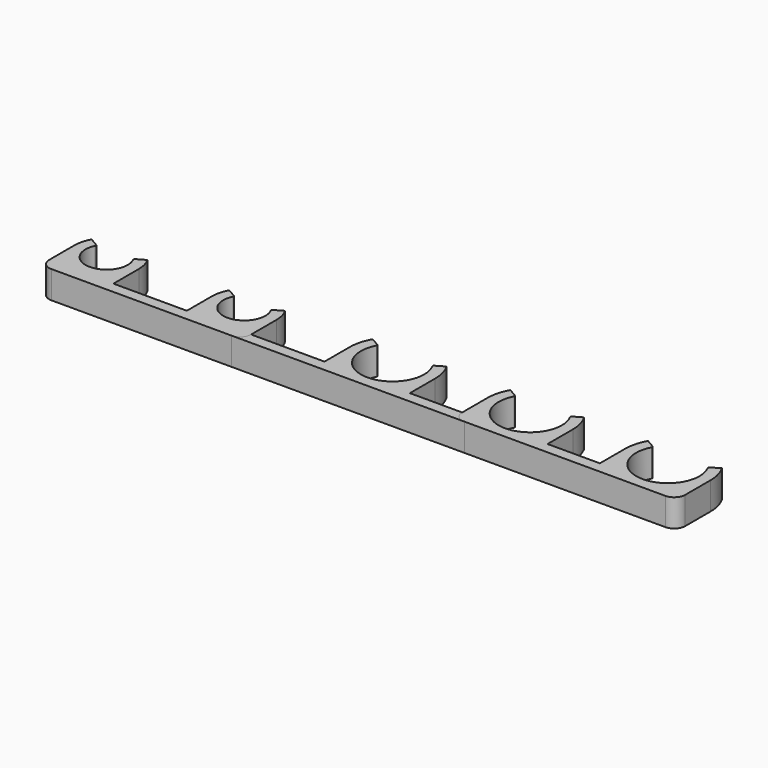
from build123d import *

# Parameters (mm, degrees)
F1_DEPTH = 5
F2_DEPTH = 5


# Not quite as in the source:
# - a feature names something its author has since deleted; it is built from what else it names


with BuildPart() as f1:
    # F0 (on Top) → F1 (new body)
    with BuildSketch(Plane.XY):
        with BuildLine():
            ThreePointArc((5.0906607601, 2.6735132364), (0, -5.75), (-5.0906607601, 2.6735132364))
            ThreePointArc((-5.0906607601, 2.6735132364), (-5.0718550548, 2.8592753519), (-5.1869938367, 3.0062592933))
            Line((-5.1869938367, 3.0062592933), (-6.7066912921, 3.8836570282))
            ThreePointArc((-6.7066912921, 3.8836570282), (-7.4846295003, 2.0106768122), (-7.75, 0))
            ThreePointArc((-7.75, 0), (-5.4800775542, -5.4800775542), (0, -7.75))
            ThreePointArc((0, -7.75), (5.4800775542, -5.4800775542), (7.75, 0))
            ThreePointArc((7.75, 0), (7.4846295003, 2.0106768122), (6.7066912921, 3.8836570282))
            Line((6.7066912921, 3.8836570282), (5.1869938367, 3.0062592933))
            ThreePointArc((5.1869938367, 3.0062592933), (5.0718550548, 2.8592753519), (5.0906607601, 2.6735132364))
        make_face()
        with BuildLine():
            ThreePointArc((0, -7.75), (-5.4800775542, -5.4800775542), (-7.75, 0))
            Line((-7.75, 0), (-7.75, -5.75))
            Line((-7.75, -5.75), (-21.075, -5.75))
            ThreePointArc((-21.075, -5.75), (-21.6607864376, -7.1642135624), (-23.075, -7.75))
            Line((-23.075, -7.75), (-7.75, -7.75))
            Line((-7.75, -7.75), (-5.75, -7.75))
            Line((-5.75, -7.75), (0, -7.75))
        make_face()
        with BuildLine():
            Line((7.75, -5.75), (7.75, 0))
            ThreePointArc((7.75, 0), (5.4800775542, -5.4800775542), (0, -7.75))
            Line((0, -7.75), (5.75, -7.75))
            Line((5.75, -7.75), (19.25, -7.75))
            ThreePointArc((19.25, -7.75), (17.8357864376, -7.1642135624), (17.25, -5.75))
            Line((17.25, -5.75), (7.75, -5.75))
        make_face()
    extrude(amount=F1_DEPTH)


with BuildPart() as f2:
    # F0 (on Top) → F2 (new body)
    with BuildSketch(Plane.XY):
        with BuildLine():
            ThreePointArc((-57.75, 0), (-51.9125, -5.8375), (-46.075, 0))
            ThreePointArc((-46.075, 0), (-46.2757134574, 1.5175782427), (-46.8640513825, 2.9307972987))
            Line((-46.8640513825, 2.9307972987), (-48.3854905692, 2.0523939747))
            ThreePointArc((-48.3854905692, 2.0523939747), (-48.5000018905, 1.9075418417), (-48.4838550604, 1.723600919))
            ThreePointArc((-48.4838550604, 1.723600919), (-51.9048651488, -3.8374924051), (-55.3479761214, 1.7099444637))
            ThreePointArc((-55.3479761214, 1.7099444637), (-55.3324173522, 1.8934720901), (-55.4467856407, 2.0378478482))
            Line((-55.4467856407, 2.0378478482), (-56.9690803045, 2.9167450821))
            ThreePointArc((-56.9690803045, 2.9167450821), (-57.5513914592, 1.5097381764), (-57.75, 0))
        make_face()
        with BuildLine():
            Line((-55.75, -7.75), (-48.075, -7.75))
            ThreePointArc((-48.075, -7.75), (-46.6607864376, -7.1642135624), (-46.075, -5.75))
            Line((-46.075, -5.75), (-46.075, 0))
            ThreePointArc((-46.075, 0), (-51.9125, -5.8375), (-57.75, 0))
            Line((-57.75, 0), (-57.75, -5.75))
            ThreePointArc((-57.75, -5.75), (-57.1642135624, -7.1642135624), (-55.75, -7.75))
        make_face()
        with BuildLine():
            ThreePointArc((-32.75, 0), (-26.9125, -5.8375), (-21.075, 0))
            ThreePointArc((-21.075, 0), (-21.2757134574, 1.5175782427), (-21.8640513825, 2.9307972987))
            Line((-21.8640513825, 2.9307972987), (-23.3854905692, 2.0523939747))
            ThreePointArc((-23.3854905692, 2.0523939747), (-23.5000018905, 1.9075418417), (-23.4838550604, 1.723600919))
            ThreePointArc((-23.4838550604, 1.723600919), (-26.9048651488, -3.8374924051), (-30.3479761214, 1.7099444637))
            ThreePointArc((-30.3479761214, 1.7099444637), (-30.3324173522, 1.8934720901), (-30.4467856407, 2.0378478482))
            Line((-30.4467856407, 2.0378478482), (-31.9690803045, 2.9167450821))
            ThreePointArc((-31.9690803045, 2.9167450821), (-32.5513914592, 1.5097381764), (-32.75, 0))
        make_face()
        with BuildLine():
            ThreePointArc((-23.075, -7.75), (-21.6607864376, -7.1642135624), (-21.075, -5.75))
            Line((-21.075, -5.75), (-21.075, 0))
            ThreePointArc((-21.075, 0), (-26.9125, -5.8375), (-32.75, 0))
            Line((-32.75, 0), (-32.75, -5.75))
            ThreePointArc((-32.75, -5.75), (-32.1642135624, -7.1642135624), (-30.75, -7.75))
            Line((-30.75, -7.75), (-23.075, -7.75))
        make_face()
        with BuildLine():
            Line((-48.075, -7.75), (-30.75, -7.75))
            ThreePointArc((-30.75, -7.75), (-32.1642135624, -7.1642135624), (-32.75, -5.75))
            Line((-32.75, -5.75), (-46.075, -5.75))
            ThreePointArc((-46.075, -5.75), (-46.6607864376, -7.1642135624), (-48.075, -7.75))
        make_face()
    extrude(amount=F2_DEPTH)


with BuildPart() as f2b:
    # F0 (on Top) → F2, piece 2 (new body)
    with BuildSketch(Plane.XY):
        with BuildLine():
            ThreePointArc((18.2933087079, 3.8836570282), (17.5153704997, 2.0106768122), (17.25, 0))
            ThreePointArc((17.25, 0), (19.5199224458, -5.4800775542), (25, -7.75))
            ThreePointArc((25, -7.75), (30.4800775542, -5.4800775542), (32.75, 0))
            ThreePointArc((32.75, 0), (32.4846295003, 2.0106768122), (31.7066912921, 3.8836570282))
            Line((31.7066912921, 3.8836570282), (30.1869938367, 3.0062592933))
            ThreePointArc((30.1869938367, 3.0062592933), (30.0718550548, 2.8592753519), (30.0906607601, 2.6735132364))
            ThreePointArc((30.0906607601, 2.6735132364), (25, -5.75), (19.9093392399, 2.6735132364))
            ThreePointArc((19.9093392399, 2.6735132364), (19.9281449452, 2.8592753519), (19.8130061633, 3.0062592933))
            Line((19.8130061633, 3.0062592933), (18.2933087079, 3.8836570282))
        make_face()
        with BuildLine():
            Line((17.25, 0), (17.25, -5.75))
            ThreePointArc((17.25, -5.75), (17.8357864376, -7.1642135624), (19.25, -7.75))
            Line((19.25, -7.75), (25, -7.75))
            ThreePointArc((25, -7.75), (19.5199224458, -5.4800775542), (17.25, 0))
        make_face()
        with BuildLine():
            ThreePointArc((32.75, 0), (30.4800775542, -5.4800775542), (25, -7.75))
            Line((25, -7.75), (30.75, -7.75))
            ThreePointArc((30.75, -7.75), (32.1642135624, -7.1642135624), (32.75, -5.75))
            Line((32.75, -5.75), (32.75, 0))
        make_face()
        with BuildLine():
            ThreePointArc((42.25, 0), (44.5199224458, -5.4800775542), (50, -7.75))
            ThreePointArc((50, -7.75), (55.4800775542, -5.4800775542), (57.75, 0))
            ThreePointArc((57.75, 0), (57.4846295003, 2.0106768122), (56.7066912921, 3.8836570282))
            Line((56.7066912921, 3.8836570282), (55.1869938367, 3.0062592933))
            ThreePointArc((55.1869938367, 3.0062592933), (55.0718550548, 2.8592753519), (55.0906607601, 2.6735132364))
            ThreePointArc((55.0906607601, 2.6735132364), (50, -5.75), (44.9093392399, 2.6735132364))
            ThreePointArc((44.9093392399, 2.6735132364), (44.9281449452, 2.8592753519), (44.8130061633, 3.0062592933))
            Line((44.8130061633, 3.0062592933), (43.2933087079, 3.8836570282))
            ThreePointArc((43.2933087079, 3.8836570282), (42.5153704997, 2.0106768122), (42.25, 0))
        make_face()
        with BuildLine():
            ThreePointArc((42.25, -5.75), (42.8357864376, -7.1642135624), (44.25, -7.75))
            Line((44.25, -7.75), (50, -7.75))
            ThreePointArc((50, -7.75), (44.5199224458, -5.4800775542), (42.25, 0))
            Line((42.25, 0), (42.25, -5.75))
        make_face()
        with BuildLine():
            ThreePointArc((57.75, 0), (55.4800775542, -5.4800775542), (50, -7.75))
            Line((50, -7.75), (55.75, -7.75))
            ThreePointArc((55.75, -7.75), (57.1642135624, -7.1642135624), (57.75, -5.75))
            Line((57.75, -5.75), (57.75, 0))
        make_face()
        with BuildLine():
            ThreePointArc((32.75, -5.75), (32.1642135624, -7.1642135624), (30.75, -7.75))
            Line((30.75, -7.75), (44.25, -7.75))
            ThreePointArc((44.25, -7.75), (42.8357864376, -7.1642135624), (42.25, -5.75))
            Line((42.25, -5.75), (32.75, -5.75))
        make_face()
    extrude(amount=F2_DEPTH)


solid = Compound([f1.part, f2.part, f2b.part])
